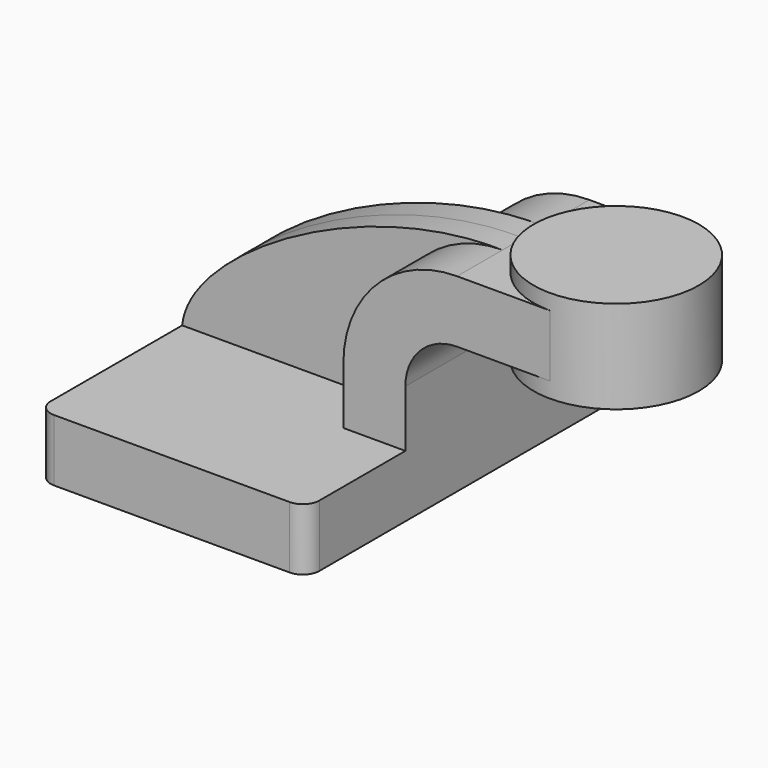
from build123d import *

# Parameters (mm, degrees)
F1_DEPTH = 63.5
F2_DEPTH = 25.4
F3_DEPTH = 7.9375
F0_W     = 25.4
F0_H     = 19.05
F4_DEPTH = 25.4
F6_R     = 5.08


# Not quite as in the source:
# - a feature names something its author has since deleted; it is built from what else it names


with BuildPart() as f1:
    # F0 (on Front) → F1 (new body, symmetric)
    with BuildSketch(Plane.XZ):
        Polygon((22.225, 9.525), (-41.275, 9.525), (-41.275, -9.525), (41.275, -9.525), (41.275, 9.525), align=None)
    extrude(amount=F1_DEPTH, both=True)

    # F0 (on Front) → F2 (join, symmetric)
    with BuildSketch(Plane.XZ):
        with BuildLine():
            Line((22.225, 27.0002), (22.225, 9.525))
            Line((22.225, 9.525), (41.275, 9.525))
            Line((41.275, 9.525), (41.275, 27.0002))
            ThreePointArc((41.275, 27.0002), (45.9246798487, 38.2255201513), (57.15, 42.8752))
            Line((57.15, 42.8752), (60.325, 42.8752))
            Line((60.325, 42.8752), (60.325, 61.9252))
            Line((60.325, 61.9252), (57.15, 61.9252))
            ThreePointArc((57.15, 61.9252), (32.4542956671, 51.6959043329), (22.225, 27.0002))
        make_face()
    extrude(amount=F2_DEPTH, both=True)

    # F0 (on Front) → F3 (join, symmetric)
    with BuildSketch(Plane.XZ):
        with BuildLine():
            add(Edge.make_bspline(
                [(-41.275, 9.525), (-39.190236479, 31.1887320131), (12.7593874931, 62.8514587879), (57.15, 61.9252)],
                knots=[0, 0, 0, 0, 111.5045361635, 111.5045361635, 111.5045361635, 111.5045361635], degree=3))
            Line((-41.275, 9.525), (22.225, 9.525))
            Line((22.225, 9.525), (22.225, 27.0002))
            ThreePointArc((22.225, 27.0002), (32.4542956671, 51.6959043329), (57.15, 61.9252))
        make_face()
    extrude(amount=F3_DEPTH, both=True)

    # F0 (on Front) → F4 (join, symmetric)
    with BuildSketch(Plane.XZ):
        with Locations((73.025, 52.4002)):
            Rectangle(F0_W, F0_H)
    extrude(amount=F4_DEPTH, both=True)

    # F0 (on Front) → F5 (revolve)
    with BuildSketch(Plane.XZ):
        Polygon((85.725, 66.675), (85.725, 61.9252), (85.725, 42.8752), (85.725, 38.1), (111.125, 38.1), (111.125, 66.675), align=None)
    revolve(axis=Axis((85.725, 0, 52.3875), (0, 0, -1)))

    # F6
    f6_edges = [f1.edges().sort_by_distance(p)[0] for p in [
        (41.275, -63.5, 0),
        (-41.275, -63.5, 0),
        (-41.275, 63.5, 0),
        (41.275, 63.5, 0),
    ]]
    fillet(f6_edges, radius=F6_R)


solid = f1.part
